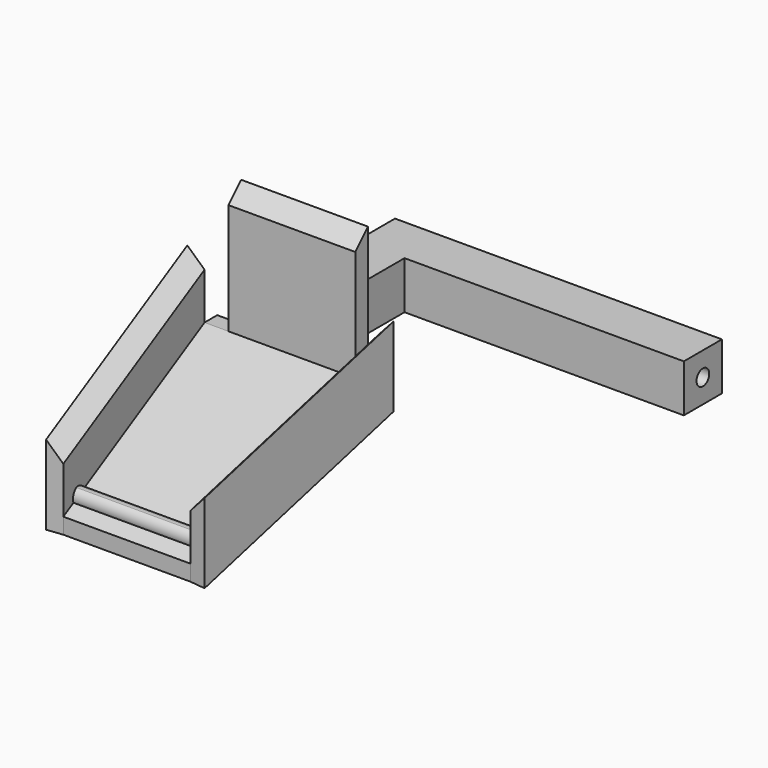
from build123d import *

# Parameters (mm, degrees)
F0_W          = 69.85
F0_H          = 6.35
F2_W          = 50.8
F2_H          = 6.35
F5_DEPTH      = 6.35
F7_DEPTH      = 6.35
F9_DEPTH      = 3.8354
F10_T4_DEPTH  = 70.8999806704
F10_T10_DEPTH = 72.2676909626
F11_W         = 69.85
F11_H         = 6.35
F12_DEPTH     = 6.35
F13_W         = 50.8
F13_H         = 6.35
F14_DEPTH     = 50.8
F15_SIZE      = 6.34999
F16_W         = 19.05
F16_H         = 19.05
F17_DEPTH     = 57.15
F18_W         = 19.05
F18_H         = 19.05
F19_DEPTH     = 111.76
F20_SIZE      = 6.34999
F21_R         = 3.175
F22_DEPTH     = 25.4


# Not quite as in the source:
# - a fillet or chamfer that OpenCascade refuses, or shapes differently, is made with other operations: its cross-section is extruded or revolved along the edge and cut away or added
# - a fillet or chamfer is up to 0.001 mm smaller than in the source, because OpenCascade refuses the exact size


with BuildPart() as f3:
    # F0 (on Front) → F3 section 0
    with BuildSketch(Plane.XZ):
        with Locations((-34.925, 3.175)):
            Rectangle(F0_W, F0_H)
    # F2 (on offset) → F3 section 1
    with BuildSketch(Plane.XZ.offset(82.55)):
        with Locations((-34.925, -28.575)):
            Rectangle(F2_W, F2_H)
    loft()

    # F4 (on face) → F5 (join)
    with BuildSketch(Plane(origin=(-68.9322627737, -7.9537226277, 0), x_dir=(0.114624108, -0.9934089359, 0), z_dir=(-0.9934089359, -0.114624108, 0))):
        Polygon((-8.0064939428, 31.75), (-8.0064939428, 6.35), (-8.0064939428, 0), (75.091208342, -31.75), (75.091208342, -25.4), (75.091208342, 0), align=None)
    extrude(amount=F5_DEPTH)

    # F6 (on face) → F7 (join)
    with BuildSketch(Plane(origin=(0, 0, 0), x_dir=(0.114624108, 0.9934089359, 0), z_dir=(0.9934089359, -0.114624108, 0))):
        Polygon((-83.0977022847, 0), (-83.0977022847, -31.75), (0, 0), (0, 31.75), align=None)
    extrude(amount=F7_DEPTH)

    # F8 (on face) → F9 (join)
    with BuildSketch(Plane(origin=(0, -2.1275773196, 5.5317010309), x_dir=(1, 0, 0), z_dir=(0, -0.3589790793, 0.9333456062))):
        Polygon((-61.6927102922, -73.4657484065), (-61.0088551461, -79.8157484065), (-8.8411448539, -79.8157484065), (-8.1572897078, -73.4657484065), align=None)
    extrude(amount=F9_DEPTH)

    # F10: fillet of radius 3.81 on 2 edges, made by hand


with BuildPart() as f10_tool2:
    # F10_s3 → F10_t4 (new body)
    with BuildSketch(Plane.YZ.offset(-70.3749903352)):
        with BuildLine():
            ThreePointArc((-76.6323734692, -23.096775868), (-76.5579487098, -20.1816780202), (-74.4440370018, -18.1730188162))
            Line((-74.4440370018, -18.1730188162), (-78.0000837614, -19.5407291084))
            Line((-78.0000837614, -19.5407291084), (-76.6323734692, -23.096775868))
        make_face()
    extrude(amount=F10_T4_DEPTH)

    split(bisect_by=Plane(origin=(0, 0, 0), x_dir=(0, 0, 1), z_dir=(-0.9934089359, 0.114624108, 0)), keep=Keep.TOP)

    split(bisect_by=Plane(origin=(-68.9322627737, -7.9537226277, 0), x_dir=(0, 0, 1), z_dir=(0.9934089359, 0.114624108, 0)), keep=Keep.TOP)


with BuildPart() as f3_1:
    add(f3.part)

    # F10_t1: cut F10_tool2
    add(f10_tool2.part, mode=Mode.SUBTRACT)


with BuildPart() as f10_tool8:
    # F10_s9 → F10_t10 (new body)
    with BuildSketch(Plane.YZ.offset(1.2088454813)):
        with BuildLine():
            ThreePointArc((-70.7056288698, -20.8172587144), (-72.7142880738, -18.7033470063), (-75.6293859216, -18.6289222469))
            Line((-75.6293859216, -18.6289222469), (-72.073339162, -17.2612119547))
            Line((-72.073339162, -17.2612119547), (-70.7056288698, -20.8172587144))
        make_face()
    extrude(amount=-F10_T10_DEPTH)

    split(bisect_by=Plane(origin=(0, 0, 0), x_dir=(0, 0, 1), z_dir=(-0.9934089359, 0.114624108, 0)), keep=Keep.TOP)

    split(bisect_by=Plane(origin=(-68.9322627737, -7.9537226277, 0), x_dir=(0, 0, 1), z_dir=(0.9934089359, 0.114624108, 0)), keep=Keep.TOP)


with BuildPart() as f3_2:
    add(f3_1.part)

    # F10_t7: cut F10_tool8
    add(f10_tool8.part, mode=Mode.SUBTRACT)

    # F11 (on face) → F12 (join)
    with BuildSketch(Plane(origin=(0, 0, 0), x_dir=(-1, 0, 0), z_dir=(0, 1, 0))):
        with Locations((34.925, 3.175)):
            Rectangle(F11_W, F11_H)
    extrude(amount=F12_DEPTH)

    # F13 (on face) → F14 (join)
    with BuildSketch(Plane.XY.offset(6.35)):
        with Locations((-34.925, 3.175)):
            Rectangle(F13_W, F13_H)
    extrude(amount=F14_DEPTH)

    # F15 (size 6.35 in the source; OpenCascade refuses exactly that, so slightly less here)
    f15_edges = [f3_2.edges().sort_by_distance(p)[0] for p in [
        (-34.925, 0, 57.15),
    ]]
    chamfer(f15_edges, length=F15_SIZE)

    # F16 (on face) → F17 (join)
    with BuildSketch(Plane(origin=(0, 6.35, 0), x_dir=(-1, 0, 0), z_dir=(0, 1, 0))):
        with Locations((34.925, 15.875)):
            Rectangle(F16_W, F16_H)
    extrude(amount=F17_DEPTH)

    # F18 (on face) → F19 (join)
    with BuildSketch(Plane.YZ.offset(-25.4)):
        with Locations((53.975, 15.875)):
            Rectangle(F18_W, F18_H)
    extrude(amount=F19_DEPTH)

    # F20 (size 6.35 in the source; OpenCascade refuses exactly that, so slightly less here)
    f20_edges = [f3_2.edges().sort_by_distance(p)[0] for p in [
        (-65.0875, -41.275, 15.875),
        (-4.7625, -41.275, 15.875),
    ]]
    chamfer(f20_edges, length=F20_SIZE)

    # F21 (on face) → F22 (cut)
    with BuildSketch(Plane.YZ.offset(86.36)):
        with Locations((53.975, 15.875)):
            Circle(F21_R)
    extrude(amount=-F22_DEPTH, mode=Mode.SUBTRACT)


solid = f3_2.part
